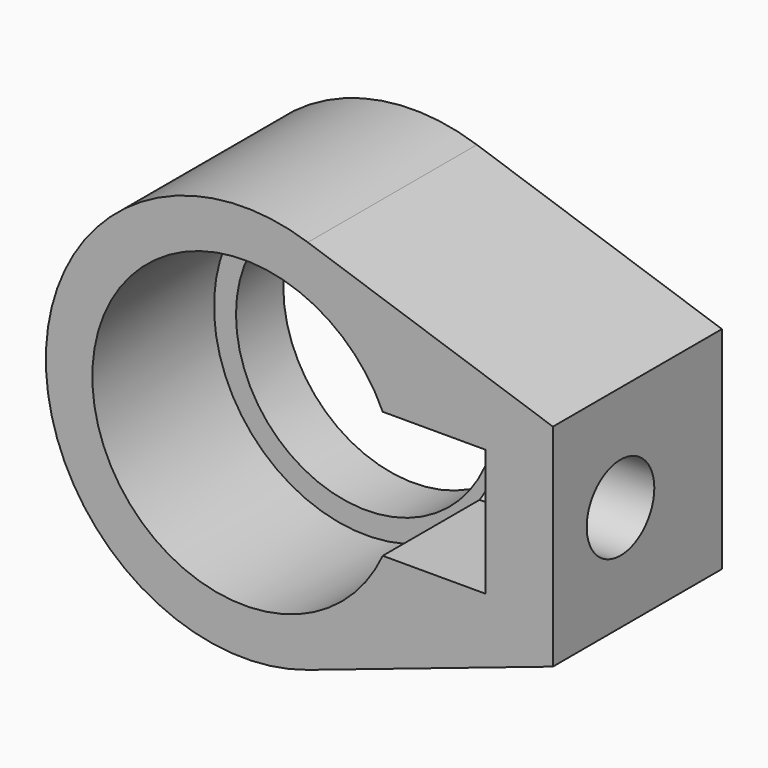
from build123d import *

# Parameters (mm, degrees)
F1_DEPTH       = 25
F2_R           = 18
F3_DEPTH       = 18
F4_R           = 15.4
F5_DEPTH       = 7
F6_R           = 5
F7_DEPTH       = 25
F9_DEPTH       = 22
F11_END_RADIUS = 18
F11_REACH      = 68.8481644957


with BuildPart() as f1:
    # F0 (on Front) → F1 (new body)
    with BuildSketch(Plane.XZ):
        with BuildLine():
            Line((60, 11), (60, 23.5))
            Line((60, 23.5), (60, 36))
            Line((60, 36), (31.0034618727, 45.7698913317))
            ThreePointArc((31.0034618727, 45.7698913317), (0, 23.5), (31.0034618727, 1.2301086683))
            Line((31.0034618727, 1.2301086683), (60, 11))
        make_face()
    extrude(amount=F1_DEPTH)

    # F2 (on face) → F3 (cut)
    with BuildSketch(Plane.XZ.offset(25)):
        with Locations((23.5, 23.5)):
            Circle(F2_R)
    extrude(amount=-F3_DEPTH, mode=Mode.SUBTRACT)

    # F4 (on face) → F5 (cut)
    with BuildSketch(Plane(origin=(0, 0, 0), x_dir=(-1, 0, 0), z_dir=(0, 1, 0))):
        with Locations((-23.5, 23.5)):
            Circle(F4_R)
    extrude(amount=-F5_DEPTH, mode=Mode.SUBTRACT)

    # F6 (on face) → F7 (cut)
    with BuildSketch(Plane.YZ.offset(60)):
        with Locations((-15, 23.5)):
            Circle(F6_R)
    extrude(amount=-F7_DEPTH, mode=Mode.SUBTRACT)

    # F8 (on face) → F9 (cut)
    with BuildSketch(Plane.XZ.offset(25)):
        with BuildLine():
            Line((52, 16), (52, 23.5))
            Line((52, 23.5), (52, 31))
            Line((52, 31), (39.863068172, 31))
            ThreePointArc((39.863068172, 31), (41.0860061852, 27.3382791004), (41.5, 23.5))
            ThreePointArc((41.5, 23.5), (41.0860061852, 19.6617208996), (39.863068172, 16))
            Line((39.863068172, 16), (52, 16))
        make_face()
    extrude(amount=-F9_DEPTH, mode=Mode.SUBTRACT)

    f11_end = (Plane(origin=(23.5, -5, 23.5), x_dir=(0, 0, -1), z_dir=(0, -1, 0)) * Cylinder(F11_END_RADIUS, 298.1207660327, mode=Mode.PRIVATE)).faces().sort_by_distance((41.5, -5, 23.5))[0]
    # F10 (on face) → F11 (join, up to the whole of a round face its end follows)
    with BuildSketch(Plane(origin=(52, 0, 0), x_dir=(0, -1, 0), z_dir=(-1, 0, 0))):
        Polygon((3, 16), (10.6698729811, 16), (6.3397459622, 23.5), (10.6698729811, 31), (3, 31), align=None)
    f11_long = extrude(amount=F11_REACH, mode=Mode.PRIVATE)
    add(split(f11_long, bisect_by=f11_end, keep=Keep.ALL, mode=Mode.PRIVATE).solids().sort_by_distance((52, -5.8943260873, 23.5))[0])


solid = f1.part
